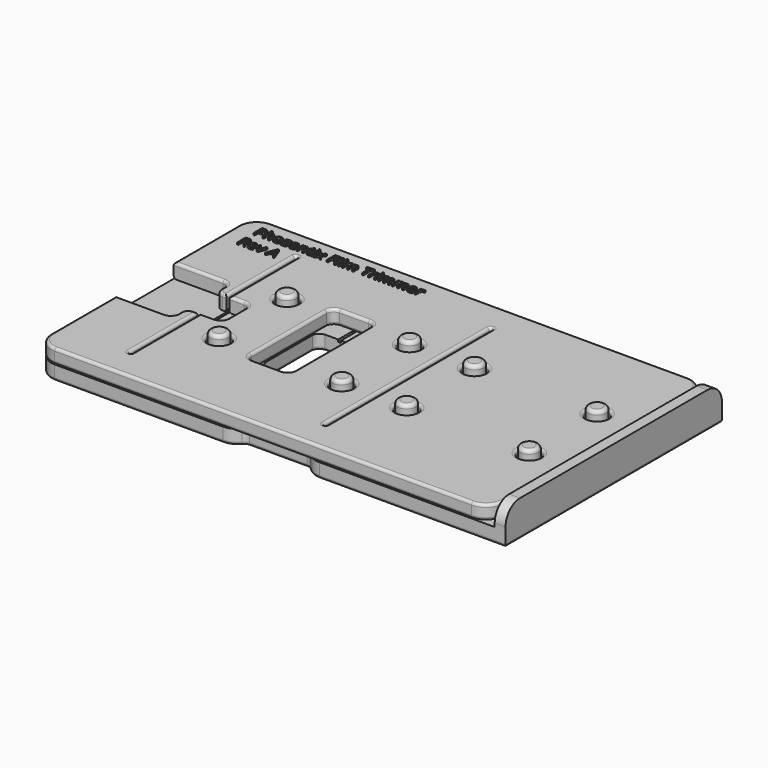
from build123d import *

# Parameters (mm, degrees)
F0_W          = 0.6
F0_H          = 58
F0_W_2        = 12
F0_H_2        = 20
F1_DEPTH      = 4
F2_R          = 2.5
F2_W          = 3
F2_H          = 75
F3_DEPTH      = 6
F4_W          = 0.8
F4_H          = 5
F5_DEPTH      = 0.6
F6_W          = 125.6017149985
F6_H          = 75
F6_R          = 3
F7_DEPTH      = 4
F8_T1_DEPTH   = 4
F9_R          = 1
F10_R         = 5
F10_2_R       = 5
F11_R         = 0.75
F12_R         = 0.75
F13_W         = 2
F13_H         = 27.885949551
F14_DEPTH     = 1
F15_R         = 3.25
F15_R_2       = 2.5
F16_DEPTH     = 0.6
F18_DEPTH     = 8.0010001
F19_T1_DEPTH  = 4
F19_T3_DEPTH  = 14.004828627
F20_R         = 0.75
F21_TEXT_SIZE = 4.1666666667
F22_DEPTH     = 0.5


# Not quite as in the source:
# - a fillet or chamfer that OpenCascade refuses, or shapes differently, is made with other operations: its cross-section is extruded or revolved along the edge and cut away or added
# - Text() gives the source's letters only with a copy of the font that has no kerning and outlines rounded to 1/6400 em; it was checked with that copy


with BuildPart() as f1:
    # F0 (on Top) → F1 (new body)
    with BuildSketch(Plane.XY):
        with BuildLine():
            Line((-10, 37.5), (-65, 37.5))
            Line((-65, 37.5), (-65, -37.5))
            Line((-65, -37.5), (-10, -37.5))
            Line((-10, -37.5), (-10, -37))
            ThreePointArc((-10, -37), (-9.4142135624, -35.5857864376), (-8, -35))
            Line((-8, -35), (8, -35))
            ThreePointArc((8, -35), (9.4142135624, -35.5857864376), (10, -37))
            Line((10, -37), (10, -37.5))
            Line((10, -37.5), (65, -37.5))
            Line((65, -37.5), (65, 37.5))
            Line((65, 37.5), (10, 37.5))
            Line((10, 37.5), (10, 37))
            ThreePointArc((10, 37), (9.4142135624, 35.5857864376), (8, 35))
            Line((8, 35), (-8, 35))
            ThreePointArc((-8, 35), (-9.4142135624, 35.5857864376), (-10, 37))
            Line((-10, 37), (-10, 37.5))
        make_face()
        with Locations((-46, 0)):
            Rectangle(F0_W, F0_H, mode=Mode.SUBTRACT)
        with Locations((-19, 0)):
            Rectangle(F0_W_2, F0_H_2, mode=Mode.SUBTRACT)
        with Locations((8, 0)):
            Rectangle(F0_W, F0_H, mode=Mode.SUBTRACT)
    extrude(amount=F1_DEPTH)

    # F2 (on face) → F3 (join)
    with BuildSketch(Plane.XY.offset(4)):
        with Locations((-35, 11.75)):
            Circle(F2_R)
        with Locations((-1, 11.75)):
            Circle(F2_R)
        with Locations((17, 11.75)):
            Circle(F2_R)
        with Locations((51, 11.75)):
            Circle(F2_R)
        with Locations((-35, -11.75)):
            Circle(F2_R)
        with Locations((-1, -11.75)):
            Circle(F2_R)
        with Locations((17, -11.75)):
            Circle(F2_R)
        with Locations((51, -11.75)):
            Circle(F2_R)
        with Locations((63.5, 0)):
            Rectangle(F2_W, F2_H)
    extrude(amount=F3_DEPTH)

    # F4 (on face) → F5 (cut)
    with BuildSketch(Plane.XY.offset(4)):
        with Locations((-19, 12.5)):
            Rectangle(F4_W, F4_H)
        with Locations((-19, -12.5)):
            Rectangle(F4_W, F4_H)
    extrude(amount=-F5_DEPTH, mode=Mode.SUBTRACT)

    # F8: fillet of radius 2 on 4 edges, made by hand

    # F8_s2 → F8_t1 (join)
    with BuildSketch(Plane.XY):
        with BuildLine():
            ThreePointArc((-25.0004, 7.9990343146), (-24.4142135624, 9.4142135624), (-22.9990343146, 10.0004))
            Line((-22.9990343146, 10.0004), (-22.9990343146, 10.2005365685))
            ThreePointArc((-22.9990343146, 10.2005365685), (-23.9995171573, 10.2001365685), (-25, 10.2001365685))
            Line((-25, 10.2001365685), (-25.2001365685, 10))
            ThreePointArc((-25.2001365685, 10), (-25.2001365685, 8.9995171573), (-25.2005365685, 7.9990343146))
            Line((-25.2005365685, 7.9990343146), (-25.0004, 7.9990343146))
        make_face()
        with BuildLine():
            ThreePointArc((-15.0009656854, 10.0004), (-13.5857864376, 9.4142135624), (-12.9996, 7.9990343146))
            Line((-12.9996, 7.9990343146), (-12.7994634315, 7.9990343146))
            ThreePointArc((-12.7994634315, 7.9990343146), (-12.7998634315, 8.9995171573), (-12.7998634315, 10))
            Line((-12.7998634315, 10), (-13, 10.2001365685))
            ThreePointArc((-13, 10.2001365685), (-14.0004828427, 10.2001365685), (-15.0009656854, 10.2005365685))
            Line((-15.0009656854, 10.2005365685), (-15.0009656854, 10.0004))
        make_face()
        with BuildLine():
            ThreePointArc((-12.9996, -7.9990343146), (-13.5857864376, -9.4142135624), (-15.0009656854, -10.0004))
            Line((-15.0009656854, -10.0004), (-15.0009656854, -10.2005365685))
            ThreePointArc((-15.0009656854, -10.2005365685), (-14.0004828427, -10.2001365685), (-13, -10.2001365685))
            Line((-13, -10.2001365685), (-12.7998634315, -10))
            ThreePointArc((-12.7998634315, -10), (-12.7998634315, -8.9995171573), (-12.7994634315, -7.9990343146))
            Line((-12.7994634315, -7.9990343146), (-12.9996, -7.9990343146))
        make_face()
        with BuildLine():
            ThreePointArc((-25.0004, -7.9990343146), (-24.4142135624, -9.4142135624), (-22.9990343146, -10.0004))
            Line((-22.9990343146, -10.0004), (-22.9990343146, -10.2005365685))
            ThreePointArc((-22.9990343146, -10.2005365685), (-23.9995171573, -10.2001365685), (-25, -10.2001365685))
            Line((-25, -10.2001365685), (-25.2001365685, -10))
            ThreePointArc((-25.2001365685, -10), (-25.2001365685, -8.9995171573), (-25.2005365685, -7.9990343146))
            Line((-25.2005365685, -7.9990343146), (-25.0004, -7.9990343146))
        make_face()
    extrude(amount=F8_T1_DEPTH)

    # F9
    f9_edges = [f1.edges().sort_by_distance(p)[0] for p in [
        (-37.5, 11.75, 10),
        (-37.5, -11.75, 10),
        (-3.5, 11.75, 10),
        (-3.5, -11.75, 10),
        (14.5, 11.75, 10),
        (14.5, -11.75, 10),
        (48.5, 11.75, 10),
        (48.5, -11.75, 10),
    ]]
    fillet(f9_edges, radius=F9_R)

    # F10
    f10_edges = [f1.edges().sort_by_distance(p)[0] for p in [
        (-65, -37.5, 2),
        (-65, 37.5, 2),
        (-10, -37.5, 2),
        (10, 37.5, 2),
        (-10, 37.5, 2),
        (63.5, 37.5, 10),
        (63.5, -37.5, 10),
        (10, -37.5, 2),
    ]]
    fillet(f10_edges, radius=F10_R)

    # F11
    f11_edges = [f1.edges().sort_by_distance(p)[0] for p in [
        (-36.680951, 37.5, 0),
        (-11.249017, 37.031635, 0),
        (-63.535534, 36.035534, 0),
        (-8.845154, 35.187346, 0),
        (-65, 0, 0),
        (0, 35, 0),
        (-63.535534, -36.035534, 0),
        (8.845154, 35.187346, 0),
        (-36.680951, -37.5, 0),
        (11.249017, 37.031635, 0),
        (-11.249017, -37.031635, 0),
        (39.180951, 37.5, 0),
        (-8.845154, -35.187346, 0),
        (65, 0, 0),
        (0, -35, 0),
        (39.180951, -37.5, 0),
        (8.845154, -35.187346, 0),
        (11.249017, -37.031635, 0),
        (-46.3, 0, 0),
        (-46, 29, 0),
        (-45.7, 0, 0),
        (-46, -29, 0),
        (-19, -10, 0),
        (-24.414214, -9.414214, 0),
        (-25, 0, 0),
        (-24.414214, 9.414214, 0),
        (-19, 10, 0),
        (-13.585786, 9.414214, 0),
        (-13, 0, 0),
        (-13.585786, -9.414214, 0),
        (7.7, 0, 0),
        (8, 29, 0),
        (8.3, 0, 0),
        (8, -29, 0),
    ]]
    fillet(f11_edges, radius=F11_R)

    # F13 (on face) → F14 (cut)
    with BuildSketch(Plane.XY.offset(4)):
        with Locations((61, 0)):
            Rectangle(F13_W, F13_H)
    extrude(amount=-F14_DEPTH, mode=Mode.SUBTRACT)

    # F15 (on face) → F16 (cut)
    with BuildSketch(Plane.XY.offset(4)):
        with Locations((-35, 11.75)):
            Circle(F15_R)
        with Locations((-35, 11.75)):
            Circle(F15_R_2, mode=Mode.SUBTRACT)
        with Locations((-1, 11.75)):
            Circle(F15_R)
        with Locations((-1, 11.75)):
            Circle(F15_R_2, mode=Mode.SUBTRACT)
        with Locations((17, 11.75)):
            Circle(F15_R)
        with Locations((17, 11.75)):
            Circle(F15_R_2, mode=Mode.SUBTRACT)
        with Locations((51, 11.75)):
            Circle(F15_R)
        with Locations((51, 11.75)):
            Circle(F15_R_2, mode=Mode.SUBTRACT)
        with Locations((-35, -11.75)):
            Circle(F15_R)
        with Locations((-35, -11.75)):
            Circle(F15_R_2, mode=Mode.SUBTRACT)
        with Locations((-1, -11.75)):
            Circle(F15_R)
        with Locations((-1, -11.75)):
            Circle(F15_R_2, mode=Mode.SUBTRACT)
        with Locations((17, -11.75)):
            Circle(F15_R)
        with Locations((17, -11.75)):
            Circle(F15_R_2, mode=Mode.SUBTRACT)
        with Locations((51, -11.75)):
            Circle(F15_R)
        with Locations((51, -11.75)):
            Circle(F15_R_2, mode=Mode.SUBTRACT)
    extrude(amount=-F16_DEPTH, mode=Mode.SUBTRACT)


with BuildPart() as f7:
    # F6 (on face) → F7 (new body)
    with BuildSketch(Plane.XY.offset(4)):
        with Locations((-2.1991425008, 0)):
            Rectangle(F6_W, F6_H)
        with Locations((-35, -11.75)):
            Circle(F6_R, mode=Mode.SUBTRACT)
        with Locations((-1, -11.75)):
            Circle(F6_R, mode=Mode.SUBTRACT)
        with Locations((17, -11.75)):
            Circle(F6_R, mode=Mode.SUBTRACT)
        with Locations((51, -11.75)):
            Circle(F6_R, mode=Mode.SUBTRACT)
        with BuildLine():
            Line((-46.4, -28.6), (-46.4, 28.6))
            ThreePointArc((-46.4, 28.6), (-46.2828427125, 28.8828427125), (-46, 29))
            ThreePointArc((-46, 29), (-45.7171572875, 28.8828427125), (-45.6, 28.6))
            Line((-45.6, 28.6), (-45.6, -28.6))
            ThreePointArc((-45.6, -28.6), (-45.7171572875, -28.8828427125), (-46, -29))
            ThreePointArc((-46, -29), (-46.2828427125, -28.8828427125), (-46.4, -28.6))
        make_face(mode=Mode.SUBTRACT)
        with Locations((-35, 11.75)):
            Circle(F6_R, mode=Mode.SUBTRACT)
        with BuildLine():
            ThreePointArc((-25, 13), (-24.4142135624, 14.4142135624), (-23, 15))
            Line((-23, 15), (-15, 15))
            ThreePointArc((-15, 15), (-13.5857864376, 14.4142135624), (-13, 13))
            Line((-13, 13), (-13, -13))
            ThreePointArc((-13, -13), (-13.5857864376, -14.4142135624), (-15, -15))
            Line((-15, -15), (-23, -15))
            ThreePointArc((-23, -15), (-24.4142135624, -14.4142135624), (-25, -13))
            Line((-25, -13), (-25, 13))
        make_face(mode=Mode.SUBTRACT)
        with BuildLine():
            Line((7.6, -28.6), (7.6, 28.6))
            ThreePointArc((7.6, 28.6), (7.7171572875, 28.8828427125), (8, 29))
            ThreePointArc((8, 29), (8.2828427125, 28.8828427125), (8.4, 28.6))
            Line((8.4, 28.6), (8.4, -28.6))
            ThreePointArc((8.4, -28.6), (8.2828427125, -28.8828427125), (8, -29))
            ThreePointArc((8, -29), (7.7171572875, -28.8828427125), (7.6, -28.6))
        make_face(mode=Mode.SUBTRACT)
        with Locations((-1, 11.75)):
            Circle(F6_R, mode=Mode.SUBTRACT)
        with Locations((17, 11.75)):
            Circle(F6_R, mode=Mode.SUBTRACT)
        with Locations((51, 11.75)):
            Circle(F6_R, mode=Mode.SUBTRACT)
    extrude(amount=F7_DEPTH)

    # F10#2
    f10_2_edges = [f7.edges().sort_by_distance(p)[0] for p in [
        (60.601715, -37.5, 6),
        (-65, 37.5, 6),
        (60.601715, 37.5, 6),
        (-65, -37.5, 6),
    ]]
    fillet(f10_2_edges, radius=F10_2_R)

    # F12
    f12_edges = [f7.edges().sort_by_distance(p)[0] for p in [
        (-2.199143, 37.5, 4),
        (59.137249, 36.035534, 4),
        (-63.535534, 36.035534, 4),
        (60.601715, 0, 4),
        (-65, 0, 4),
        (59.137249, -36.035534, 4),
        (-63.535534, -36.035534, 4),
        (-2.199143, -37.5, 4),
        (-38, -11.75, 4),
        (-4, -11.75, 4),
        (14, -11.75, 4),
        (48, -11.75, 4),
        (-46.4, 0, 4),
        (-46, 29, 4),
        (-45.6, 0, 4),
        (-46, -29, 4),
        (-38, 11.75, 4),
        (-24.414214, 14.414214, 4),
        (-19, 15, 4),
        (-13.585786, 14.414214, 4),
        (-13, 0, 4),
        (-13.585786, -14.414214, 4),
        (-19, -15, 4),
        (-24.414214, -14.414214, 4),
        (-25, 0, 4),
        (8, -29, 4),
        (7.6, 0, 4),
        (8, 29, 4),
        (8.4, 0, 4),
        (-4, 11.75, 4),
        (14, 11.75, 4),
        (48, 11.75, 4),
    ]]
    fillet(f12_edges, radius=F12_R)

    # F17 (on face) → F18 (cut, through all)
    with BuildSketch(Plane.XY.offset(8)):
        Polygon((-39.5941626419, 5), (-49.4, 5), (-49.4, 10), (-65, 10), (-65, -10), (-49.4, -10), (-49.4, -5), (-39.5941626419, -5), align=None)
    extrude(amount=-F18_DEPTH, mode=Mode.SUBTRACT)

    # F19: fillet of radius 2 on 6 edges, made by hand

    # F19_s2 → F19_t1 (join)
    with BuildSketch(Plane.XY.offset(4)):
        with BuildLine():
            ThreePointArc((-39.5937626419, 2.9990343146), (-40.1799490796, 4.4142135624), (-41.5951283274, 5.0004))
            Line((-41.5951283274, 5.0004), (-41.5951283274, 5.2005365685))
            ThreePointArc((-41.5951283274, 5.2005365685), (-40.5946454847, 5.2001365685), (-39.5941626419, 5.2001365685))
            Line((-39.5941626419, 5.2001365685), (-39.3940260734, 5))
            ThreePointArc((-39.3940260734, 5), (-39.3940260734, 3.9995171573), (-39.3936260734, 2.9990343146))
            Line((-39.3936260734, 2.9990343146), (-39.5937626419, 2.9990343146))
        make_face()
        with BuildLine():
            ThreePointArc((-41.5951283274, -5.0004), (-40.1799490796, -4.4142135624), (-39.5937626419, -2.9990343146))
            Line((-39.5937626419, -2.9990343146), (-39.3936260734, -2.9990343146))
            ThreePointArc((-39.3936260734, -2.9990343146), (-39.3940260734, -3.9995171573), (-39.3940260734, -5))
            Line((-39.3940260734, -5), (-39.5941626419, -5.2001365685))
            ThreePointArc((-39.5941626419, -5.2001365685), (-40.5946454847, -5.2001365685), (-41.5951283274, -5.2005365685))
            Line((-41.5951283274, -5.2005365685), (-41.5951283274, -5.0004))
        make_face()
        with BuildLine():
            ThreePointArc((-49.3996, 7.9990343146), (-49.9857864376, 9.4142135624), (-51.4009656854, 10.0004))
            Line((-51.4009656854, 10.0004), (-51.4009656854, 10.2005365685))
            ThreePointArc((-51.4009656854, 10.2005365685), (-50.4004828427, 10.2001365685), (-49.4, 10.2001365685))
            Line((-49.4, 10.2001365685), (-49.1998634315, 10))
            ThreePointArc((-49.1998634315, 10), (-49.1998634315, 8.9995171573), (-49.1994634315, 7.9990343146))
            Line((-49.1994634315, 7.9990343146), (-49.3996, 7.9990343146))
        make_face()
        with BuildLine():
            ThreePointArc((-51.4009656854, -10.0004), (-49.9857864376, -9.4142135624), (-49.3996, -7.9990343146))
            Line((-49.3996, -7.9990343146), (-49.1994634315, -7.9990343146))
            ThreePointArc((-49.1994634315, -7.9990343146), (-49.1998634315, -8.9995171573), (-49.1998634315, -10))
            Line((-49.1998634315, -10), (-49.4, -10.2001365685))
            ThreePointArc((-49.4, -10.2001365685), (-50.4004828427, -10.2001365685), (-51.4009656854, -10.2005365685))
            Line((-51.4009656854, -10.2005365685), (-51.4009656854, -10.0004))
        make_face()
    extrude(amount=F19_T1_DEPTH)

    # F19_s4 → F19_t3 (cut)
    with BuildSketch(Plane.XY.offset(-1.0024143135)):
        with BuildLine():
            ThreePointArc((-49.4004, -7.0009656854), (-48.8142135624, -5.5857864376), (-47.3990343146, -4.9996))
            Line((-47.3990343146, -4.9996), (-47.3990343146, -4.7994634315))
            ThreePointArc((-47.3990343146, -4.7994634315), (-48.3995171573, -4.7998634315), (-49.4, -4.7998634315))
            Line((-49.4, -4.7998634315), (-49.6001365685, -5))
            ThreePointArc((-49.6001365685, -5), (-49.6001365685, -6.0004828427), (-49.6005365685, -7.0009656854))
            Line((-49.6005365685, -7.0009656854), (-49.4004, -7.0009656854))
        make_face()
        with BuildLine():
            ThreePointArc((-47.3990343146, 4.9996), (-48.8142135624, 5.5857864376), (-49.4004, 7.0009656854))
            Line((-49.4004, 7.0009656854), (-49.6005365685, 7.0009656854))
            ThreePointArc((-49.6005365685, 7.0009656854), (-49.6001365685, 6.0004828427), (-49.6001365685, 5))
            Line((-49.6001365685, 5), (-49.4, 4.7998634315))
            ThreePointArc((-49.4, 4.7998634315), (-48.3995171573, 4.7998634315), (-47.3990343146, 4.7994634315))
            Line((-47.3990343146, 4.7994634315), (-47.3990343146, 4.9996))
        make_face()
    extrude(amount=F19_T3_DEPTH, mode=Mode.SUBTRACT)

    # F20
    f20_edges = [f7.edges().sort_by_distance(p)[0] for p in [
        (59.137249, 36.035534, 8),
        (60.601715, 0, 8),
        (59.137249, -36.035534, 8),
        (-2.199143, -37.5, 8),
        (-63.535534, -36.035534, 8),
        (-65, -21.25, 8),
        (-58.180477, -10, 8),
        (-49.985786, -9.414214, 8),
        (-49.4, -7.5, 8),
        (-48.814214, -5.585786, 8),
        (-46.919523, -5, 8),
        (-46.4, -16.8, 8),
        (-46, -29, 8),
        (-45.6, -16.8, 8),
        (-43.577558, -5, 8),
        (-40.179949, -4.414214, 8),
        (-39.594163, 0, 8),
        (-40.179949, 4.414214, 8),
        (-43.577558, 5, 8),
        (-45.6, 16.8, 8),
        (-46, 29, 8),
        (-46.4, 16.8, 8),
        (-46.919523, 5, 8),
        (-48.814214, 5.585786, 8),
        (-49.4, 7.5, 8),
        (-49.985786, 9.414214, 8),
        (-58.180477, 10, 8),
        (-65, 21.25, 8),
        (-63.535534, 36.035534, 8),
        (-2.199143, 37.5, 8),
        (-38, -11.75, 8),
        (-4, -11.75, 8),
        (14, -11.75, 8),
        (48, -11.75, 8),
        (-24.414214, 14.414214, 8),
        (-25, 0, 8),
        (-19, 15, 8),
        (-24.414214, -14.414214, 8),
        (-13.585786, 14.414214, 8),
        (-19, -15, 8),
        (-13, 0, 8),
        (-13.585786, -14.414214, 8),
        (-38, 11.75, 8),
        (-4, 11.75, 8),
        (8, -29, 8),
        (7.6, 0, 8),
        (8.4, 0, 8),
        (8, 29, 8),
        (14, 11.75, 8),
        (48, 11.75, 8),
    ]]
    fillet(f20_edges, radius=F20_R)

    # F21 (on face) → F22 (join)
    with BuildSketch(Plane.XY.offset(8)):
        with Locations((-59.9112504165, 30.804005747)):
            Text('Phosentix Film Trimmer', F21_TEXT_SIZE, font='Open Sans', text_align=(TextAlign.LEFT, TextAlign.BOTTOM))
        with Locations((-59.9112504165, 25.1373390804)):
            Text('Rev A', F21_TEXT_SIZE, font='Open Sans', text_align=(TextAlign.LEFT, TextAlign.BOTTOM))
    extrude(amount=F22_DEPTH)


solid = Compound([f1.part, f7.part])
